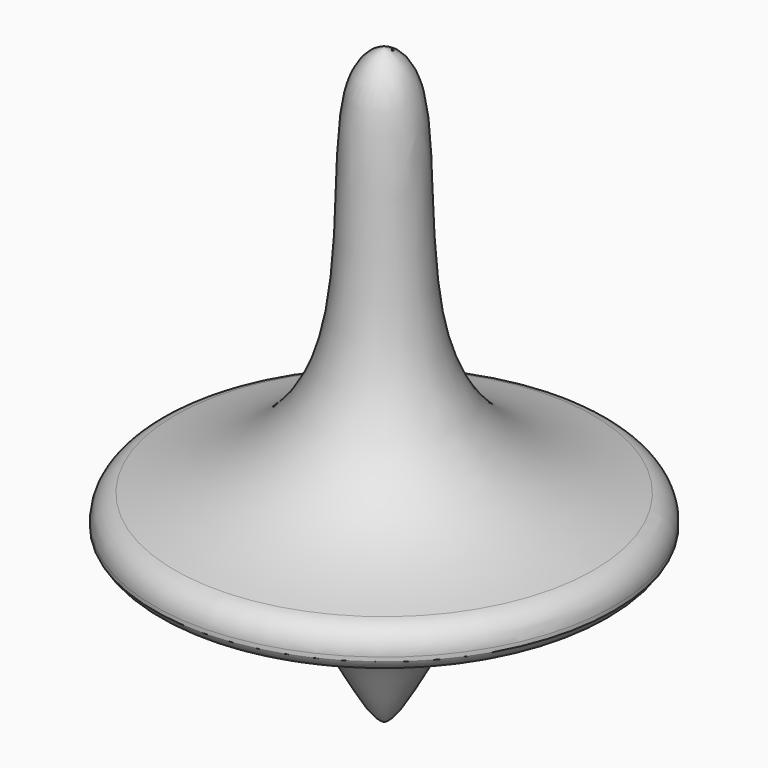
from build123d import *


# Not quite as in the source:
# - a fillet or chamfer that OpenCascade refuses, or shapes differently, is made with other operations: its cross-section is extruded or revolved along the edge and cut away or added


with BuildPart() as f1:
    # F0 (on Front) → F1 (revolve)
    with BuildSketch(Plane.XZ):
        with BuildLine():
            Line((0, 33), (0, 0))
            Line((0, 0), (18, 0))
            Line((18, 0), (18, 2))
            add(Edge.make_bspline(
                [(18, 2), (15.8767193278, 2.2997949203), (11.3169572026, 3.5400315099), (6.936903079, 6.6058969156), (3.2799320985, 12.4102253579), (2.9476917719, 23.598533786), (2.6811530149, 32.3646539521), (0, 33)],
                knots=[0, 0, 0, 0, 0.1873001398, 0.3513331882, 0.5318184857, 0.7827778744, 1, 1, 1, 1], degree=3))
        make_face()
    revolve(axis=Axis((0, 0, 16.5), (0, 0, 1)))

    # F4: fillet of radius 2 on 1 edges, made by hand

    # F4_s1 → F4_t2 (revolve, cut)
    with BuildSketch(Plane.XZ):
        with BuildLine():
            ThreePointArc((18, 0.3228205545), (17.5526182459, 1.5835253505), (16.4106234174, 2.2802138234))
            Line((16.4106234174, 2.2802138234), (16.4188358857, 2.3193616887))
            ThreePointArc((16.4188358857, 2.3193616887), (17.2099496362, 2.1663384242), (18.0055922997, 2.0396071481))
            Line((18.0055922997, 2.0396071481), (18.04, 2))
            Line((18.04, 2), (18.04, 0.3228205545))
            Line((18.04, 0.3228205545), (18, 0.3228205545))
        make_face()
    revolve(axis=Axis((0, 0, 2), (0, 0, 1)), mode=Mode.SUBTRACT)


with BuildPart() as f3:
    # F2 (on Front) → F3 (revolve)
    with BuildSketch(Plane.XZ):
        with BuildLine():
            Line((18, 0), (0, 0))
            Line((0, 0), (0, -13.5))
            add(Edge.make_bspline(
                [(0, -13.5), (0.3537948145, -13.4052397407), (1.4715501043, -12.1117596027), (3.428359406, -8.101125754), (7.3765069909, -2.5539137252), (14.7296146505, -1.1124110975), (18, -1)],
                knots=[0, 0, 0, 0, 0.1423784213, 0.3722917637, 0.6506734348, 1, 1, 1, 1], degree=3))
            Line((18, -1), (18, 0))
        make_face()
    revolve(axis=Axis((0, 0, -6.75), (0, 0, -1)))

    # F4#2: fillet of radius 2 on 1 edges, made by hand

    # F4_2_s1 → F4_2_t2 (revolve, cut)
    with BuildSketch(Plane.XZ):
        with BuildLine():
            ThreePointArc((16.3976778659, -1.1053556528), (17.3423919425, -0.7607720845), (18, 0))
            Line((18, 0), (18.035865739, -0.0177101316))
            ThreePointArc((18.035865739, -0.0177101316), (18.04, -0.5), (18.04, -1))
            Line((18.04, -1), (18.0013740858, -1.0399763916))
            ThreePointArc((18.0013740858, -1.0399763916), (17.2006681044, -1.0803582257), (16.4014971623, -1.1451728975))
            Line((16.4014971623, -1.1451728975), (16.3976778659, -1.1053556528))
        make_face()
    revolve(axis=Axis((0, 0, -1), (0, 0, -1)), mode=Mode.SUBTRACT)


solid = Compound([f1.part, f3.part])
